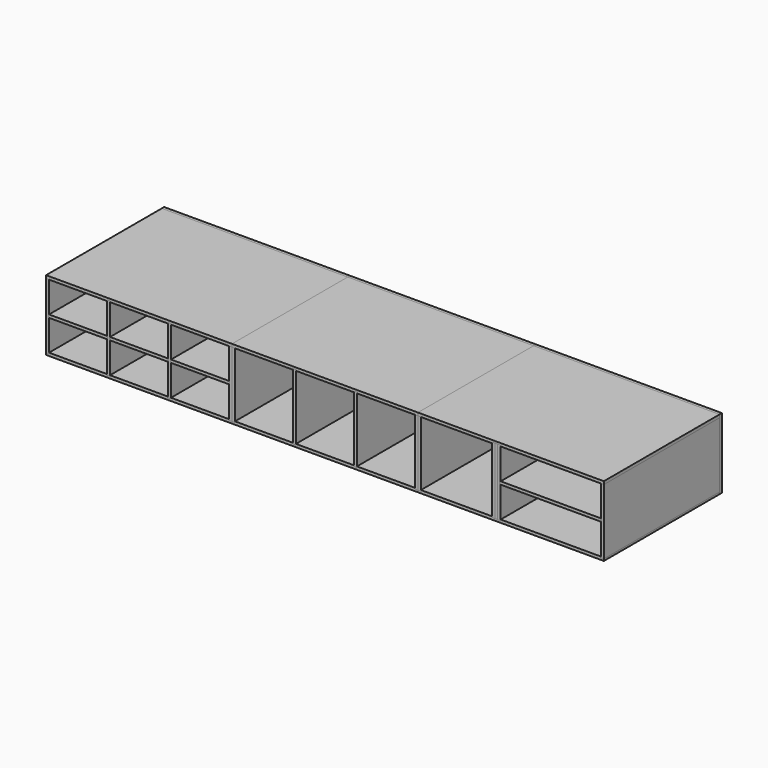
from build123d import *

# Parameters (mm, degrees)
F2_W           = 1143
F2_H           = 889
F3_DEPTH       = 18.25625
F4_DEPTH       = 18.25625
F5_DEPTH       = 18.25625
F6_W           = 18.25625
F6_H           = 889
F7_DEPTH       = 401.6375
F7_DEPTH_BACK  = 6.35
F8_W           = 18.25625
F8_H           = 889
F9_DEPTH       = 401.6375
F9_DEPTH_BACK  = 6.35
F12_W          = 18.25625
F12_H          = 889
F13_DEPTH      = 401.6375
F13_DEPTH_BACK = 6.35
F14_W          = 363.0083333333
F14_H          = 18.25625
F15_DEPTH      = 889
F14_W_2        = 359.8333333333
F16_DEPTH      = 3.175
F17_W          = 18.25625
F17_H          = 889
F18_DEPTH      = 401.6375
F18_DEPTH_BACK = 6.35
F19_W          = 18.25625
F19_H          = 889
F20_DEPTH      = 401.6375
F20_DEPTH_BACK = 6.35
F23_W          = 18.25625
F23_H          = 889
F24_DEPTH      = 401.6375
F24_DEPTH_BACK = 6.35
F25_W          = 18.25625
F25_H          = 889
F26_DEPTH      = 401.6375
F26_DEPTH_BACK = 6.35
F27_DEPTH      = 401.6375
F27_DEPTH_BACK = 6.35
F29_W          = 18.25625
F29_H          = 889
F30_DEPTH      = 401.6375
F30_DEPTH_BACK = 6.35
F31_DEPTH      = 401.6375
F31_DEPTH_BACK = 6.35
F32_DEPTH      = 401.6375
F32_DEPTH_BACK = 6.35
F33_W          = 889
F33_H          = 18.25625
F34_DEPTH      = 615.95
F35_DEPTH      = 6.35
F36_DEPTH      = 3.175
F37_W          = 1143
F37_H          = 18.25625
F37_H_2        = 413.54375
F38_DEPTH      = 18.25625
F39_DEPTH      = 18.25625
F37_H_3        = 431.8
F40_DEPTH      = 18.25625


# Not quite as in the source:
# - a length typed as a fraction of an inch, garbled in the dataset ("3 / 203.2 mm" for 3/8 in), is restored


with BuildPart() as f3:
    # F2 (on Top) → F3 (new body)
    with BuildSketch(Plane.XY):
        with Locations((571.5, -444.5)):
            Rectangle(F2_W, F2_H)
    extrude(amount=F3_DEPTH)


with BuildPart() as f4:
    # F2 (on Top) → F4 (new body)
    with BuildSketch(Plane.XY):
        with Locations((1714.5, -444.5)):
            Rectangle(F2_W, F2_H)
    extrude(amount=F4_DEPTH)


with BuildPart() as f5:
    # F2 (on Top) → F5 (new body)
    with BuildSketch(Plane.XY):
        with Locations((2857.5, -444.5)):
            Rectangle(F2_W, F2_H)
    extrude(amount=F5_DEPTH)


with BuildPart() as f7:
    # F6 (on face) → F7 (new body, two sides)
    with BuildSketch(Plane.XY.offset(18.25625)) as f7_sk:
        with Locations((1133.871875, -444.5)):
            Rectangle(F6_W, F6_H)
    extrude(amount=F7_DEPTH)
    extrude(f7_sk.sketch, amount=-F7_DEPTH_BACK)


with BuildPart() as f9:
    # F8 (on face) → F9 (new body, two sides)
    with BuildSketch(Plane.XY.offset(18.25625)) as f9_sk:
        with Locations((9.128125, -444.5)):
            Rectangle(F8_W, F8_H)
    extrude(amount=F9_DEPTH)
    extrude(f9_sk.sketch, amount=-F9_DEPTH_BACK)


with BuildPart() as f10_1:
    # F10: copy of F3
    add(f3.part.moved(Location((0, 0, 413.54375))))


with BuildPart() as f13:
    # F12 (on face) → F13 (new body, two sides)
    with BuildSketch(Plane.XY.offset(18.25625)) as f13_sk:
        with Locations((758.9572916667, -444.5)):
            Rectangle(F12_W, F12_H)
    extrude(amount=F13_DEPTH)
    extrude(f13_sk.sketch, amount=-F13_DEPTH_BACK)


with BuildPart() as f13b:
    # F12 (on face) → F13, piece 2 (new body, two sides)
    with BuildSketch(Plane.XY.offset(18.25625)) as f13_2_sk:
        with Locations((384.0427083333, -444.5)):
            Rectangle(F12_W, F12_H)
    extrude(amount=F13_DEPTH)
    extrude(f13_2_sk.sketch, amount=-F13_DEPTH_BACK)


with BuildPart() as f15:
    # F14 (on face) → F15 (new body, through all)
    with BuildSketch(Plane(origin=(0, 0, 0), x_dir=(-1, 0, 0), z_dir=(0, 1, 0))):
        with Locations((-196.5854166667, 215.9)):
            Rectangle(F14_W, F14_H)
    extrude(amount=-F15_DEPTH)


with BuildPart() as f15b:
    # F14 (on face) → F15, piece 2 (new body, through all)
    with BuildSketch(Plane(origin=(0, 0, 0), x_dir=(-1, 0, 0), z_dir=(0, 1, 0))):
        with Locations((-571.5, 215.9)):
            Rectangle(F14_W, F14_H)
    extrude(amount=-F15_DEPTH)


with BuildPart() as f15c:
    # F14 (on face) → F15, piece 3 (new body, through all)
    with BuildSketch(Plane(origin=(0, 0, 0), x_dir=(-1, 0, 0), z_dir=(0, 1, 0))):
        with Locations((-944.8270833333, 215.9)):
            Rectangle(F14_W_2, F14_H)
    extrude(amount=-F15_DEPTH)

    # F16 (add): a face of the model
    f16_faces = [f15c.faces().sort_by_distance(p)[0] for p in [
        (1124.74375, -444.5, 215.9),
    ]]
    extrude(f16_faces, amount=F16_DEPTH)


with BuildPart() as f18:
    # F17 (on face) → F18 (new body, two sides)
    with BuildSketch(Plane.XY.offset(18.25625)) as f18_sk:
        with Locations((1152.128125, -444.5)):
            Rectangle(F17_W, F17_H)
    extrude(amount=F18_DEPTH)
    extrude(f18_sk.sketch, amount=-F18_DEPTH_BACK)


with BuildPart() as f20:
    # F19 (on face) → F20 (new body, two sides)
    with BuildSketch(Plane.XY.offset(18.25625)) as f20_sk:
        with Locations((2276.871875, -444.5)):
            Rectangle(F19_W, F19_H)
    extrude(amount=F20_DEPTH)
    extrude(f20_sk.sketch, amount=-F20_DEPTH_BACK)


with BuildPart() as f21_1:
    # F21: copy of F4
    add(f4.part.moved(Location((0, 0, 413.54375))))


with BuildPart() as f24:
    # F23 (on face) → F24 (new body, two sides)
    with BuildSketch(Plane.XY.offset(18.25625)) as f24_sk:
        with Locations((1527.0427083333, -444.5)):
            Rectangle(F23_W, F23_H)
    extrude(amount=F24_DEPTH)
    extrude(f24_sk.sketch, amount=-F24_DEPTH_BACK)


with BuildPart() as f24b:
    # F23 (on face) → F24, piece 2 (new body, two sides)
    with BuildSketch(Plane.XY.offset(18.25625)) as f24_2_sk:
        with Locations((1901.9572916667, -444.5)):
            Rectangle(F23_W, F23_H)
    extrude(amount=F24_DEPTH)
    extrude(f24_2_sk.sketch, amount=-F24_DEPTH_BACK)


with BuildPart() as f26:
    # F25 (on face) → F26 (new body, two sides)
    with BuildSketch(Plane.XY.offset(18.25625)) as f26_sk:
        with Locations((2295.128125, -444.5)):
            Rectangle(F25_W, F25_H)
    extrude(amount=F26_DEPTH)
    extrude(f26_sk.sketch, amount=-F26_DEPTH_BACK)


with BuildPart() as f27:
    # F25 (on face) → F27 (new body, two sides)
    with BuildSketch(Plane.XY.offset(18.25625)) as f27_sk:
        with Locations((2295.128125, -444.5)):
            Rectangle(F25_W, F25_H)
    extrude(amount=F27_DEPTH)
    extrude(f27_sk.sketch, amount=-F27_DEPTH_BACK)


with BuildPart() as f27b:
    # F25 (on face) → F27, piece 2 (new body, two sides)
    with BuildSketch(Plane.XY.offset(18.25625)) as f27_2_sk:
        with Locations((3419.871875, -444.5)):
            Rectangle(F25_W, F25_H)
    extrude(amount=F27_DEPTH)
    extrude(f27_2_sk.sketch, amount=-F27_DEPTH_BACK)


with BuildPart() as f28_1:
    # F28: copy of F5
    add(f5.part.moved(Location((0, 0, 413.54375))))


with BuildPart() as f30:
    # F29 (on face) → F30 (new body, two sides)
    with BuildSketch(Plane.XY.offset(18.25625)) as f30_sk:
        with Locations((2785.665625, -444.5)):
            Rectangle(F29_W, F29_H)
    extrude(amount=F30_DEPTH)
    extrude(f30_sk.sketch, amount=-F30_DEPTH_BACK)


with BuildPart() as f31:
    # F29 (on face) → F31 (new body, two sides)
    with BuildSketch(Plane.XY.offset(18.25625)) as f31_sk:
        with Locations((2767.409375, -444.5)):
            Rectangle(F29_W, F29_H)
    extrude(amount=F31_DEPTH)
    extrude(f31_sk.sketch, amount=-F31_DEPTH_BACK)


with BuildPart() as f32:
    # F29 (on face) → F32 (new body, two sides)
    with BuildSketch(Plane.XY.offset(18.25625)) as f32_sk:
        with Locations((2749.153125, -444.5)):
            Rectangle(F29_W, F29_H)
    extrude(amount=F32_DEPTH)
    extrude(f32_sk.sketch, amount=-F32_DEPTH_BACK)


with BuildPart() as f34:
    # F33 (on face) → F34 (new body, through all)
    with BuildSketch(Plane.YZ.offset(2794.79375)):
        with Locations((-444.5, 215.9)):
            Rectangle(F33_W, F33_H)
    extrude(amount=F34_DEPTH)

    # F33 (on face) → F35 (join)
    with BuildSketch(Plane.YZ.offset(2794.79375)):
        with Locations((-444.5, 215.9)):
            Rectangle(F33_W, F33_H)
    extrude(amount=-F35_DEPTH)

    # F36 (add): a face of the model
    f36_faces = [f34.faces().sort_by_distance(p)[0] for p in [
        (3410.74375, -444.5, 215.9),
    ]]
    extrude(f36_faces, amount=F36_DEPTH)


with BuildPart() as f38:
    # F37 (on face) → F38 (new body)
    with BuildSketch(Plane(origin=(0, 0, 0), x_dir=(-1, 0, 0), z_dir=(0, 1, 0))):
        with Locations((-2857.5, 422.671875)):
            Rectangle(F37_W, F37_H)
        with Locations((-2857.5, 206.771875)):
            Rectangle(F37_W, F37_H_2)
    extrude(amount=F38_DEPTH)


with BuildPart() as f39:
    # F37 (on face) → F39 (new body)
    with BuildSketch(Plane(origin=(0, 0, 0), x_dir=(-1, 0, 0), z_dir=(0, 1, 0))):
        Polygon((-2286, 0), (-1143, 0), (-1143, 431.8), (-2286, 431.8), (-2286, 413.54375), align=None)
    extrude(amount=F39_DEPTH)


with BuildPart() as f40:
    # F37 (on face) → F40 (new body)
    with BuildSketch(Plane(origin=(0, 0, 0), x_dir=(-1, 0, 0), z_dir=(0, 1, 0))):
        with Locations((-571.5, 215.9)):
            Rectangle(F37_W, F37_H_3)
    extrude(amount=F40_DEPTH)


solid = Compound([f3.part, f4.part, f5.part, f7.part, f9.part, f10_1.part, f13.part, f13b.part, f15.part, f15b.part, f15c.part, f18.part, f20.part, f21_1.part, f24.part, f24b.part, f26.part, f27.part, f27b.part, f28_1.part, f30.part, f31.part, f32.part, f34.part, f38.part, f39.part, f40.part])
